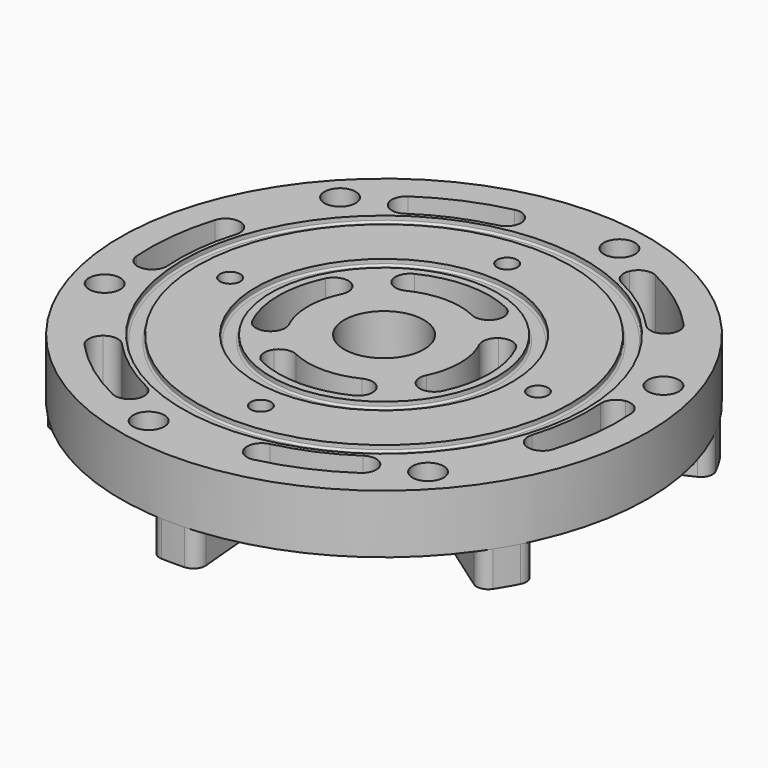
from build123d import *

# Parameters (mm, degrees)
F0_R             = 57.15
F1_DEPTH         = 12.7
F2_R             = 8.636
F3_DEPTH         = 12.701
F5_DEPTH         = 7.62
F6_T1_DEPTH      = 14.2671475518
F6_T3_DEPTH      = 13.7344913133
F8_COUNT         = 6
F9_D             = 4.3942
F9_DEPTH         = 15.24
F9_TIP           = 1.3201508661
F10_R            = 43.6245
F10_R_2          = 40.4241
F11_DEPTH        = 1.2954
F12_R            = 0.4064
F14_DEPTH        = 20.321
F14_COPIES_COUNT = 6
F15_R            = 3.17499
F16_R            = 27.7495
F16_R_2          = 24.5491
F17_DEPTH        = 1.2954
F18_R            = 0.4064
F20_DEPTH        = 20.321
F20_COPIES_COUNT = 4
F21_R            = 3.17499
F23_D            = 4.3942
F23_DEPTH        = 6.35
F23_TIP          = 1.3201508661
F25_D            = 6.7564


# Not quite as in the source:
# - a fillet or chamfer that OpenCascade refuses, or shapes differently, is made with other operations: its cross-section is extruded or revolved along the edge and cut away or added
# - a fillet or chamfer is up to 0.001 mm smaller than in the source, because OpenCascade refuses the exact size
# - a pattern or mirror of a feature is missing from the dataset's text; its kind, count and spacing are read off the source's solid


with BuildPart() as f1:
    # F0 (on Top) → F1 (new body)
    with BuildSketch(Plane.XY):
        Circle(F0_R)
    extrude(amount=F1_DEPTH)

    # F2 (on face) → F3 (cut, through all)
    with BuildSketch(Plane.XY.offset(12.7)):
        Circle(F2_R)
    extrude(amount=-F3_DEPTH, mode=Mode.SUBTRACT)

    # F4 (on face) → F5 (join)
    with BuildSketch(Plane(origin=(0, 0, 0), x_dir=(1, 0, 0), z_dir=(0, 0, -1))):
        with BuildLine():
            Line((-2.8575, -31.6211510504), (-5.1435, -56.9180718907))
            ThreePointArc((-5.1435, -56.9180718907), (0, -57.15), (5.1435, -56.9180718907))
            Line((5.1435, -56.9180718907), (2.8575, -31.6211510504))
            ThreePointArc((2.8575, -31.6211510504), (0, -31.75), (-2.8575, -31.6211510504))
        make_face()
    extrude(amount=F5_DEPTH)

    # F6: fillet of radius 2.54 on 4 edges, made by hand

    # F6_s2 → F6_t1 (cut)
    with BuildSketch(Plane.XY.offset(-14.2671475518)):
        with BuildLine():
            ThreePointArc((2.490581259, 57.0957047858), (4.2919178251, 56.2301660065), (4.9095808426, 54.3295179065))
            Line((4.9095808426, 54.3295179065), (5.1435, 56.9180718907))
            ThreePointArc((5.1435, 56.9180718907), (3.8180737982, 57.022318547), (2.490581259, 57.0957047858))
        make_face()
        with BuildLine():
            ThreePointArc((-2.490581259, 57.0957047858), (-4.2919178251, 56.2301660065), (-4.9095808426, 54.3295179065))
            Line((-4.9095808426, 54.3295179065), (-5.1435, 56.9180718907))
            ThreePointArc((-5.1435, 56.9180718907), (-3.8180737982, 57.022318547), (-2.490581259, 57.0957047858))
        make_face()
    extrude(amount=F6_T1_DEPTH, mode=Mode.SUBTRACT)

    # F6_s4 → F6_t3 (cut)
    with BuildSketch(Plane.XY.offset(-13.7344913133)):
        with BuildLine():
            ThreePointArc((0.5073422252, 31.7459462588), (2.2462164703, 32.396860006), (3.0776216873, 34.0570219595))
            Line((3.0776216873, 34.0570219595), (2.8575, 31.6211510504))
            ThreePointArc((2.8575, 31.6211510504), (1.6835778156, 31.7053318188), (0.5073422252, 31.7459462588))
        make_face()
        with BuildLine():
            ThreePointArc((-3.0776216873, 34.0570219595), (-2.2462164703, 32.396860006), (-0.5073422252, 31.7459462588))
            ThreePointArc((-0.5073422252, 31.7459462588), (-1.6835778156, 31.7053318188), (-2.8575, 31.6211510504))
            Line((-2.8575, 31.6211510504), (-3.0776216873, 34.0570219595))
        make_face()
    extrude(amount=F6_T3_DEPTH, mode=Mode.SUBTRACT)

    # F8: F1 ×6 about axis
    f8_axis = Axis((0, 0, 12.7), (0, 0, 1))


with BuildPart() as f1_1:
    add(f1.part)
    for i in range(1, F8_COUNT):
        add(f1.part.rotate(f8_axis, i * 360 / F8_COUNT))

    # F9
    with Locations(Plane(origin=(0, 0, -7.62), x_dir=(1, 0, 0), z_dir=(0, 0, -1))):
        with Locations((0, -50.8), (43.9940905122, -25.4), (43.9940905122, 25.4), (0, 50.8), (-43.9940905122, 25.4), (-43.9940905122, -25.4)):
            Hole(F9_D / 2, depth=F9_DEPTH)
            with Locations((0, 0, -(F9_DEPTH + F9_TIP / 2))):  # 118° drill point
                Cone(0, F9_D / 2, F9_TIP, mode=Mode.SUBTRACT)

    # F10 (on face) → F11 (cut)
    with BuildSketch(Plane.XY.offset(12.7)):
        Circle(F10_R)
        Circle(F10_R_2, mode=Mode.SUBTRACT)
    extrude(amount=-F11_DEPTH, mode=Mode.SUBTRACT)

    # F12
    f12_edges = [f1_1.edges().sort_by_distance(p)[0] for p in [
        (-43.6245, 0, 11.4046),
        (-40.4241, 0, 11.4046),
    ]]
    fillet(f12_edges, radius=F12_R)

    # F13 (on face) → F14 (cut, through all)
    with BuildSketch(Plane.XY.offset(12.7)):
        with BuildLine():
            ThreePointArc((16.721010174, 41.1850739803), (26.4387827868, 35.7322440487), (34.49502146, 28.0338365993))
            Line((34.49502146, 28.0338365993), (39.4228816685, 32.0386703992))
            ThreePointArc((39.4228816685, 32.0386703992), (30.2157517563, 40.8368503413), (19.1097259131, 47.0686559775))
            Line((19.1097259131, 47.0686559775), (16.721010174, 41.1850739803))
        make_face()
    f14 = extrude(amount=-F14_DEPTH, mode=Mode.SUBTRACT)

    # F14_copies: F14 ×6 about axis
    f14_copies_axis = Axis((0, 0, 0), (0, 0, 1))
    for i in range(1, F14_COPIES_COUNT):
        add(f14.rotate(f14_copies_axis, i * 360 / F14_COPIES_COUNT), mode=Mode.SUBTRACT)

    # F15 (radius 3.175 in the source; OpenCascade refuses exactly that, so slightly less here)
    f15_edges = [f1_1.edges().sort_by_distance(p)[0] for p in [
        (39.422882, 32.03867, 6.35),
        (19.109726, 47.068656, 6.35),
        (16.72101, 41.185074, 6.35),
        (34.495021, 28.033837, 6.35),
    ]]
    fillet(f15_edges, radius=F15_R)

    # F16 (on face) → F17 (cut)
    with BuildSketch(Plane.XY.offset(12.7)):
        Circle(F16_R)
        Circle(F16_R_2, mode=Mode.SUBTRACT)
    extrude(amount=-F17_DEPTH, mode=Mode.SUBTRACT)

    # F18
    f18_edges = [f1_1.edges().sort_by_distance(p)[0] for p in [
        (-27.7495, 0, 11.4046),
        (-24.5491, 0, 11.4046),
    ]]
    fillet(f18_edges, radius=F18_R)

    # F19 (on face) → F20 (cut, through all)
    with BuildSketch(Plane.XY.offset(12.7)):
        with BuildLine():
            Line((13.111957335, -18.7258157324), (9.4697469642, -13.5242002512))
            ThreePointArc((9.4697469642, -13.5242002512), (0, -16.51), (-9.4697469642, -13.5242002512))
            Line((-9.4697469642, -13.5242002512), (-13.111957335, -18.7258157324))
            ThreePointArc((-13.111957335, -18.7258157324), (0, -22.86), (13.111957335, -18.7258157324))
        make_face()
    f20 = extrude(amount=-F20_DEPTH, mode=Mode.SUBTRACT)

    # F20_copies: F20 ×4 about axis
    f20_copies_axis = Axis((0, 0, 0), (0, 0, 1))
    for i in range(1, F20_COPIES_COUNT):
        add(f20.rotate(f20_copies_axis, i * 360 / F20_COPIES_COUNT), mode=Mode.SUBTRACT)

    # F21 (radius 3.175 in the source; OpenCascade refuses exactly that, so slightly less here)
    f21_edges = [f1_1.edges().sort_by_distance(p)[0] for p in [
        (-9.469747, -13.5242, 6.35),
        (-13.111957, -18.725816, 6.35),
        (9.469747, -13.5242, 6.35),
        (13.111957, -18.725816, 6.35),
        (-13.5242, -9.469747, 6.35),
        (-18.725816, -13.111957, 6.35),
        (-13.5242, 9.469747, 6.35),
        (-18.725816, 13.111957, 6.35),
        (13.5242, 9.469747, 6.35),
        (18.725816, 13.111957, 6.35),
        (18.725816, -13.111957, 6.35),
        (13.5242, -9.469747, 6.35),
        (-9.469747, 13.5242, 6.35),
        (-13.111957, 18.725816, 6.35),
        (13.111957, 18.725816, 6.35),
        (9.469747, 13.5242, 6.35),
        (-16.72101, -41.185074, 6.35),
        (-19.109726, -47.068656, 6.35),
        (-39.422882, -32.03867, 6.35),
        (-34.495021, -28.033837, 6.35),
        (27.306815, -35.073357, 6.35),
        (31.207789, -40.083836, 6.35),
        (8.034862, -50.160552, 6.35),
        (7.030504, -43.890483, 6.35),
        (44.027825, 6.111717, 6.35),
        (50.317515, 6.98482, 6.35),
        (47.457743, -18.121882, 6.35),
        (41.525525, -15.856647, 6.35),
        (-44.027825, -6.111717, 6.35),
        (-50.317515, -6.98482, 6.35),
        (-47.457743, 18.121882, 6.35),
        (-41.525525, 15.856647, 6.35),
        (-27.306815, 35.073357, 6.35),
        (-31.207789, 40.083836, 6.35),
        (-8.034862, 50.160552, 6.35),
        (-7.030504, 43.890483, 6.35),
    ]]
    fillet(f21_edges, radius=F21_R)

    # F23
    with Locations(Plane.XY.offset(12.7)):
        with Locations((-33.3375, 0), (0, -33.3375), (33.3375, 0), (0, 33.3375)):
            Hole(F23_D / 2, depth=F23_DEPTH)
            with Locations((0, 0, -(F23_DEPTH + F23_TIP / 2))):  # 118° drill point
                Cone(0, F23_D / 2, F23_TIP, mode=Mode.SUBTRACT)

    # F25 (through all)
    with Locations(Plane.XY.offset(12.7)):
        with Locations((11.3576544358, 49.5140756323), (48.5592745603, 14.9210205473), (37.2016201245, -34.593055085), (-11.3576544358, -49.5140756323), (-48.5592745603, -14.9210205473), (-37.2016201245, 34.593055085)):
            Hole(F25_D / 2)


solid = f1_1.part
